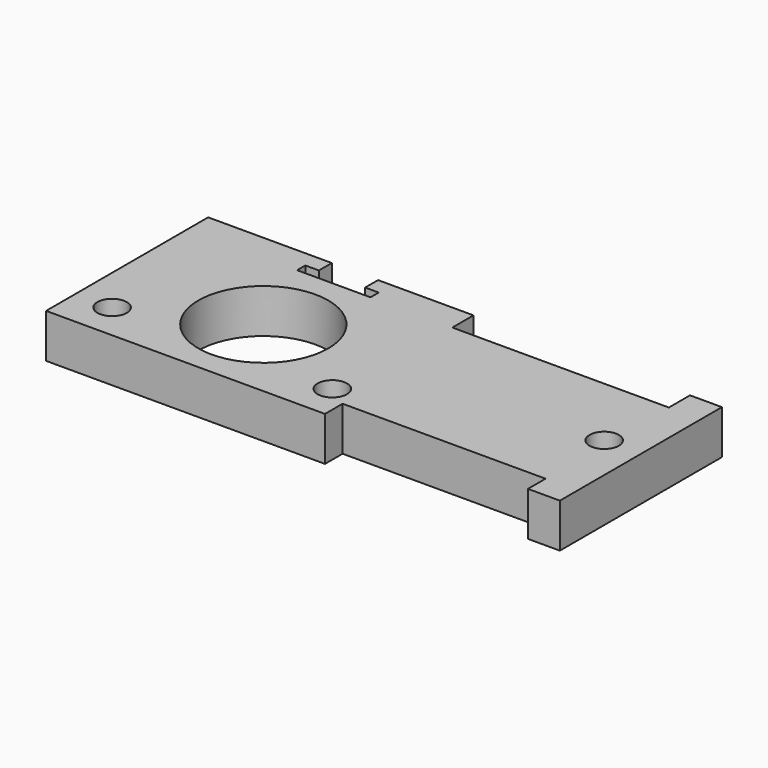
from build123d import *

# Parameters (mm, degrees)
F0_R     = 2
F0_R_2   = 8.85
F1_DEPTH = 6


# Not quite as in the source:
# - a feature names something its author has since deleted; it is built from what else it names


with BuildPart() as f1:
    # F0 (on Top) → F1 (new body)
    with BuildSketch(Plane.XY):
        Polygon((-20, 15.6), (-20, 12), (-20, -12), (18, -12), (18, -9), (45.65, -9), (45.65, -12), (50, -12), (50, 15.6), (45.65, 15.6), (45.65, 12), (16.15, 12), (16.15, 15.6), (3.15, 15.6), (3.15, 13.4), (5, 13.4), (5, 12), (-5, 12), (-5, 13.4), (-3.15, 13.4), (-3.15, 15.6), align=None)
        with Locations((-15, -7)):
            Circle(F0_R, mode=Mode.SUBTRACT)
        Circle(F0_R_2, mode=Mode.SUBTRACT)
        with Locations((15, -7)):
            Circle(F0_R, mode=Mode.SUBTRACT)
        with Locations((45, 1.8)):
            Circle(F0_R, mode=Mode.SUBTRACT)
    extrude(amount=F1_DEPTH)


solid = f1.part
